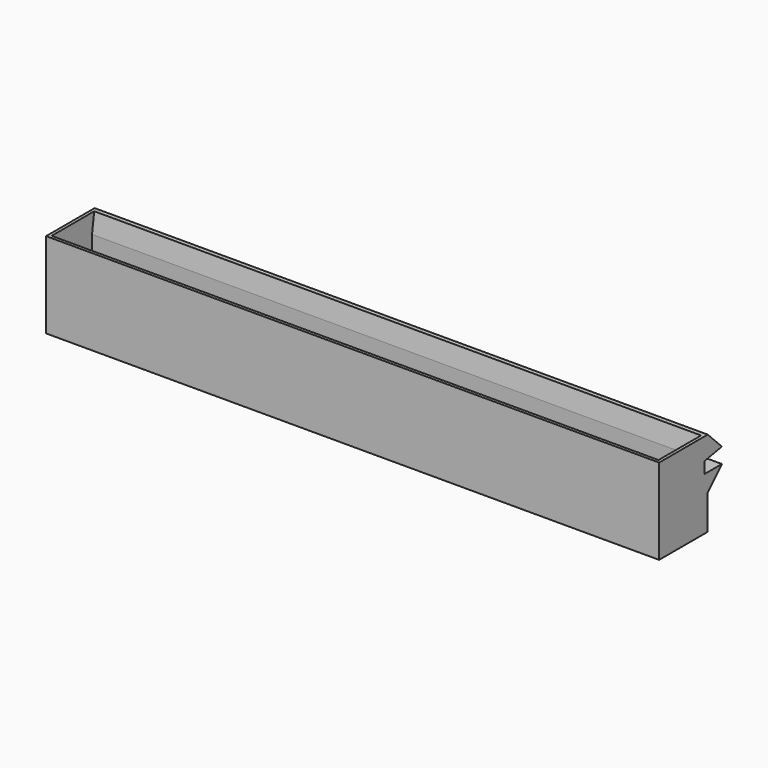
from build123d import *

# Parameters (mm, degrees)
F1_DEPTH = 100
F2_T     = -1
F4_DEPTH = 198


with BuildPart() as f1:
    # F0 (on Right) → F1 (new body, symmetric)
    with BuildSketch(Plane.YZ):
        Polygon((5.8090751991, 1.8115955126), (0, 1.8115955126), (-1.3203158755, 1.8115955126), (-1.3203158755, 0.5179099389), align=None)
        Polygon((-1.3203158755, 1.8115955126), (0, 1.8115955126), (5.8090751991, 1.8115955126), (0, 7.6206707116), (-19.7975447644, 7.6206707116), (-19.7975447644, -20.3238854808), (0, -20.3238854808), (0, -8.9974796865), (0, -3.1884044874), (-1.3203158755, -3.1884044874), (-1.3203158755, 0.5179099389), align=None)
        Polygon((5.8090751991, -3.1884044874), (0, -3.1884044874), (0, -8.9974796865), align=None)
    extrude(amount=F1_DEPTH, both=True)

    # F2
    f2_openings = [f1.faces().sort_by_distance(p)[0] for p in [
        (0, -9.898772, 7.620671),
    ]]
    offset(amount=F2_T, openings=f2_openings, kind=Kind.INTERSECTION)

    # F3 (on face) → F4 (join, through all)
    with BuildSketch(Plane.YZ.offset(-99)):
        Polygon((-1.4142135624, 7.6206707116), (-2.3203158755, 1.3527820438), (3.7518344093, 2.4546227399), align=None)
        Polygon((3.3948616367, -4.1884044874), (-2.3203158755, -4.1884044874), (-1, -8.5832661241), align=None)
    extrude(amount=F4_DEPTH)


solid = f1.part
